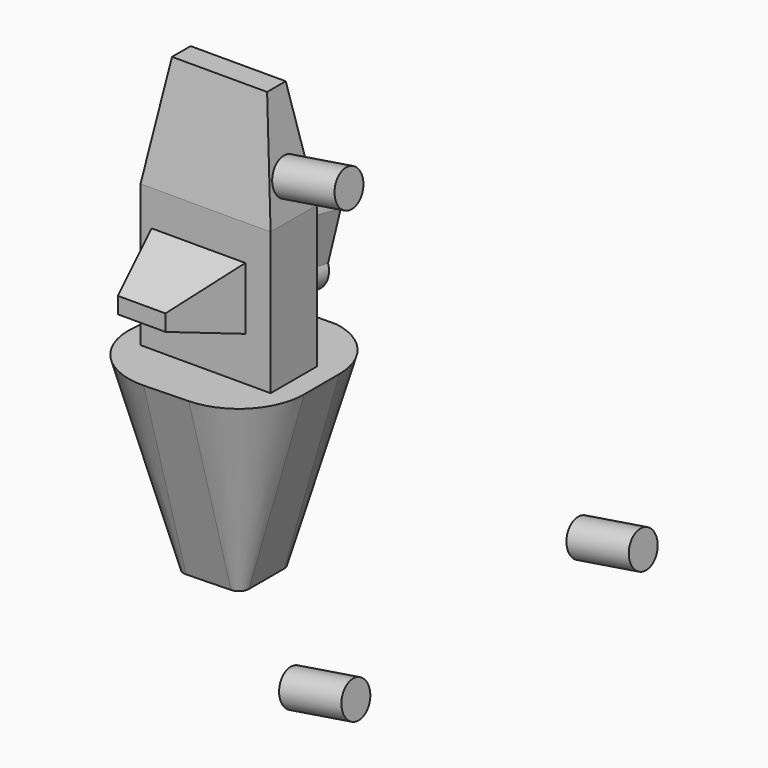
from build123d import *

# Parameters (mm, degrees)
F1_DEPTH               = 1219.2
DRAFT_F1_DRAFTED_ANGLE = -16.25
F2_W                   = 837.9063606262
F2_H                   = 375.194311142
F3_DEPTH               = 914.4
F5_DEPTH               = 304.8
DRAFT_F5_DRAFTED_ANGLE = -16
F6_W                   = 603.8489341736
F6_H                   = 402.0335674286
F7_DEPTH               = 457.2
DRAFT_F7_DRAFTED_ANGLE = 18
F3_FACE3_W             = 837.9063606262
F3_FACE3_H             = 375.194311142
F10_DEPTH              = 711.2
F10_TAPER              = 9
F11_R                  = 114.3
F12_DEPTH              = 406.4


# Not quite as in the source:
# - an extrude with a draft is written as a straight extrude whose walls are then drafted
# - the program builds the solid bodies; features that only make, move or delete a surface that nothing else refers to are left out


with BuildPart() as f1:
    # F0 (on Top) → F1 (new body)
    with BuildSketch(Plane.XY):
        with BuildLine():
            Line((239.664465772, 62.3088084797), (-43.6895745996, 58.3547787348))
            ThreePointArc((-43.6895745996, 58.3547787348), (-86.6617471987, 41.3071425033), (-107.4210703373, 0))
            Line((-107.4210703373, 0), (-136.2694759938, -281.9094110476))
            ThreePointArc((-136.2694759938, -281.9094110476), (-119.1726861202, -332.8146033284), (-69.6037791468, -353.467987714))
            Line((-69.6037791468, -353.467987714), (213.6398386548, -344.6249384213))
            ThreePointArc((213.6398386548, -344.6249384213), (258.2683315927, -324.9031069188), (276.5879064914, -279.6809199387))
            Line((276.5879064914, -279.6809199387), (276.5879064914, 3.7007071053))
            ThreePointArc((276.5879064914, 3.7007071053), (266.5874584571, 38.3354079892), (239.664465772, 62.3088084797))
        make_face()
    extrude(amount=F1_DEPTH)

    # draft_F1_drafted
    draft_f1_drafted_walls = [f1.faces().sort_by_distance(p)[0] for p in [
        (97.9874455862, 60.3317936072, 812.8),
        (-86.6617471987, 41.3071425033, 812.8),
        (-121.8452731655, -140.9547055238, 812.8),
        (-119.1726861202, -332.8146033284, 812.8),
        (72.018029754, -349.0464630676, 812.8),
        (258.2683315927, -324.9031069188, 812.8),
        (276.5879064914, -137.9901064167, 812.8),
        (266.5874584571, 38.3354079892, 812.8),
    ]]
    draft(draft_f1_drafted_walls, neutral_plane=Plane.XY, angle=DRAFT_F1_DRAFTED_ANGLE)

    # F2 (on face) → F3 (join)
    with BuildSketch(Plane.XY.offset(1219.2)):
        with Locations((73.450088501, -187.597155571)):
            Rectangle(F2_W, F2_H)
    extrude(amount=F3_DEPTH)


with BuildPart() as f5_drafted:
    # F4 (on face) → F5 (new body)
    with BuildSketch(Plane(origin=(0, 0, 0), x_dir=(-1, 0, 0), z_dir=(0, 1, 0))):
        with BuildLine():
            Line((-172.0291376114, 1516.5997743607), (68.4726238251, 1516.5997743607))
            ThreePointArc((68.4726238251, 1516.5997743607), (120.4513427915, 1552.3921030414), (105.5543422699, 1613.7187480927))
            Line((105.5543422699, 1613.7187480927), (126.0375976562, 1967.099070549))
            ThreePointArc((126.0375976562, 1967.099070549), (105.7683073659, 2041.7470739283), (35.6281995773, 2074.3589401245))
            Line((35.6281995773, 2074.3589401245), (-218.0485129356, 2074.3589401245))
            ThreePointArc((-218.0485129356, 2074.3589401245), (-287.4436301456, 2044.732189428), (-314.044713974, 1974.121928215))
            Line((-314.044713974, 1974.121928215), (-226.9156575203, 1616.5456771851))
            ThreePointArc((-226.9156575203, 1616.5456771851), (-229.0416659694, 1550.3343989074), (-172.0291376114, 1516.5997743607))
        make_face()
    extrude(amount=F5_DEPTH)

    # draft_F5_drafted
    draft_f5_drafted_walls = [f5_drafted.faces().sort_by_distance(p)[0] for p in [
        (-105.7683073659, 203.2, 2041.7470739283),
        (91.2101566792, 203.2, 2074.3589401245),
        (287.4436301456, 203.2, 2044.732189428),
        (270.4801857471, 203.2, 1795.3338027),
        (229.0416659694, 203.2, 1550.3343989074),
        (51.7782568932, 203.2, 1516.5997743607),
        (-120.4513427915, 203.2, 1552.3921030414),
        (-115.7959699631, 203.2, 1790.4089093208),
    ]]
    draft(draft_f5_drafted_walls, neutral_plane=Plane(origin=(0, 0, 0), x_dir=(-1, 0, 0), z_dir=(0, 1, 0)), angle=DRAFT_F5_DRAFTED_ANGLE)


with BuildPart() as f1_1:
    add(f1.part)

    # join_F5_drafted: union F5_drafted
    add(f5_drafted.part)


with BuildPart() as f7_drafted:
    # F6 (on face) → F7 (new body)
    with BuildSketch(Plane.XZ.offset(375.194311142)):
        with Locations((27.5337696075, 1703.70054245)):
            Rectangle(F6_W, F6_H)
    extrude(amount=F7_DEPTH)

    # draft_F7_drafted
    draft_f7_drafted_walls = [f7_drafted.faces().sort_by_distance(p)[0] for p in [
        (27.5337696075, -679.994311142, 1502.6837587357),
        (329.4582366943, -679.994311142, 1703.70054245),
        (27.5337696075, -679.994311142, 1904.7173261642),
        (-274.3906974792, -679.994311142, 1703.70054245),
    ]]
    draft(draft_f7_drafted_walls, neutral_plane=Plane.XZ.offset(375.194311142), angle=DRAFT_F7_DRAFTED_ANGLE)


with BuildPart() as f1_2:
    add(f1_1.part)

    # join_F7_drafted: union F7_drafted
    add(f7_drafted.part)

    # F3_face3 (on face) → F10 (join)
    with BuildSketch(Plane(origin=(73.450088501, -187.597155571, 2133.6), x_dir=(1, 0, 0), z_dir=(0, 0, 1))):
        Rectangle(F3_FACE3_W, F3_FACE3_H)
    extrude(amount=F10_DEPTH, taper=F10_TAPER)


with BuildPart() as f12:
    # F11 (on face) → F12 (new body)
    with BuildSketch(Plane(origin=(810.0126327316, 0, 128.293397491), x_dir=(0, 1, 0), z_dir=(0.9876883406, 0, 0.156434465))):
        with Locations((-200.3535628319, 2264.5592689514)):
            Circle(F11_R)
    extrude(amount=F12_DEPTH)


with BuildPart() as f12b:
    # F11 (on face) → F12, piece 2 (new body)
    with BuildSketch(Plane(origin=(810.0126327316, 0, 128.293397491), x_dir=(0, 1, 0), z_dir=(0.9876883406, 0, 0.156434465))):
        with Locations((1642.2974756485, -428.2327797749)):
            Circle(F11_R)
    extrude(amount=F12_DEPTH)


with BuildPart() as f12c:
    # F11 (on face) → F12, piece 3 (new body)
    with BuildSketch(Plane(origin=(810.0126327316, 0, 128.293397491), x_dir=(0, 1, 0), z_dir=(0.9876883406, 0, 0.156434465))):
        with Locations((-655.6406597553, -347.8888882219)):
            Circle(F11_R)
    extrude(amount=F12_DEPTH)


solid = Compound([f1_2.part, f12.part, f12b.part, f12c.part])
